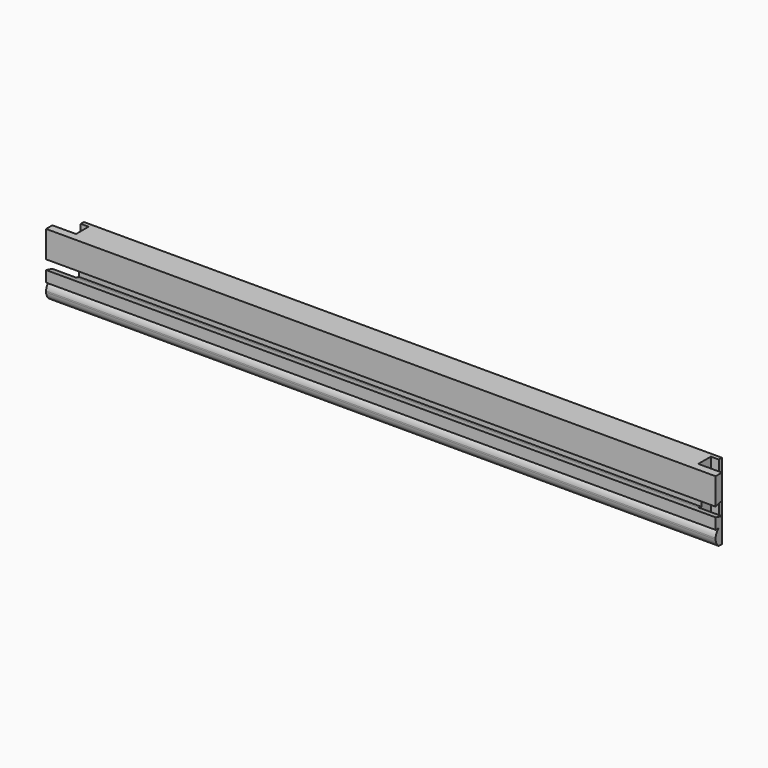
from build123d import *

# Parameters (mm, degrees)
F0_W      = 269.875
F0_H      = 11.1125
F1_DEPTH  = 25.4
F2_W      = 6.35
F2_H      = 25.4
F3_DEPTH  = 9.525
F4_DEPTH  = 6.35
F5_W      = 1.5875
F5_H      = 25.4
F6_DEPTH  = 6.35
F5_W_2    = 6.35
F7_DEPTH  = 9.525
F8_W      = 4.7625
F8_H      = 0.396875
F9_DEPTH  = 269.876
F11_DEPTH = 269.876
F12_DEPTH = 269.875
F13_DEPTH = 269.876


with BuildPart() as f1:
    # F0 (on Top) → F1 (new body)
    with BuildSketch(Plane.XY):
        with Locations((0, -5.55625)):
            Rectangle(F0_W, F0_H)
    extrude(amount=F1_DEPTH)

    # F2 (on face) → F3 (cut)
    with BuildSketch(Plane.YZ.offset(134.9375)):
        with Locations((-4.7625, 12.7)):
            Rectangle(F2_W, F2_H)
    extrude(amount=-F3_DEPTH, mode=Mode.SUBTRACT)

    # F4 (cut): a face of the model
    f4_faces = [f1.faces().sort_by_distance(p)[0] for p in [
        (134.9375, -0.79375, 12.7),
    ]]
    extrude(f4_faces, amount=-F4_DEPTH, mode=Mode.SUBTRACT)

    # F5 (on face) → F6 (cut)
    with BuildSketch(Plane(origin=(-134.9375, 0, 0), x_dir=(0, -1, 0), z_dir=(-1, 0, 0))):
        with Locations((0.79375, 12.7)):
            Rectangle(F5_W, F5_H)
    extrude(amount=-F6_DEPTH, mode=Mode.SUBTRACT)

    # F5 (on face) → F7 (cut)
    with BuildSketch(Plane(origin=(-134.9375, 0, 0), x_dir=(0, -1, 0), z_dir=(-1, 0, 0))):
        with Locations((4.7625, 12.7)):
            Rectangle(F5_W_2, F5_H)
    extrude(amount=-F7_DEPTH, mode=Mode.SUBTRACT)

    # F8 (on face) → F9 (cut, through all)
    with BuildSketch(Plane.YZ.offset(134.9375)):
        with Locations((-2.38125, 4.1671875)):
            Rectangle(F8_W, F8_H)
    extrude(amount=-F9_DEPTH, mode=Mode.SUBTRACT)

    # F10 (on face) → F11 (cut, through all)
    with BuildSketch(Plane.YZ.offset(134.9375)):
        with BuildLine():
            ThreePointArc((-9.5324710518, 0), (-10.6448555046, 1.2920515481), (-11.1125, 2.931595692))
            Line((-11.1125, 2.931595692), (-11.1125, 0))
            Line((-11.1125, 0), (-9.5324710518, 0))
        make_face()
        with BuildLine():
            Line((-11.1125, 3.418404308), (-11.1125, 6.35))
            Line((-11.1125, 6.35), (-11.1199710518, 6.35))
            Line((-11.1199710518, 6.35), (-11.1199710518, 3.175))
            ThreePointArc((-11.1199710518, 3.175), (-11.1181028492, 3.2967594696), (-11.1125, 3.418404308))
        make_face()
    extrude(amount=-F11_DEPTH, mode=Mode.SUBTRACT)

    # F10 (on face) → F12 (cut, through all)
    with BuildSketch(Plane.YZ.offset(134.9375)):
        with BuildLine():
            ThreePointArc((-11.1125, 3.418404308), (-10.6448555046, 5.0579484519), (-9.5324710518, 6.35))
            Line((-9.5324710518, 6.35), (-11.1125, 6.35))
            Line((-11.1125, 6.35), (-11.1125, 3.418404308))
        make_face()
    extrude(amount=-F12_DEPTH, mode=Mode.SUBTRACT)

    # F10 (on face) → F13 (cut, through all)
    with BuildSketch(Plane.YZ.offset(134.9375)):
        Polygon((-11.1125, 12.7), (-11.1125, 10.7991061667), (-7.9375, 9.9483674807), (-7.9375, 12.7), align=None)
        Polygon((-7.9375, 12.7), (-7.9375, 9.9483674807), (-6.3574710518, 9.525), (-6.3574710518, 12.7), align=None)
        Polygon((-11.1125, 14.6008938333), (-11.1125, 12.7), (-7.9375, 12.7), (-7.9375, 15.4516325193), align=None)
        Polygon((-7.9375, 15.4516325193), (-7.9375, 12.7), (-6.3574710518, 12.7), (-6.3574710518, 15.875), align=None)
    extrude(amount=-F13_DEPTH, mode=Mode.SUBTRACT)


solid = f1.part
